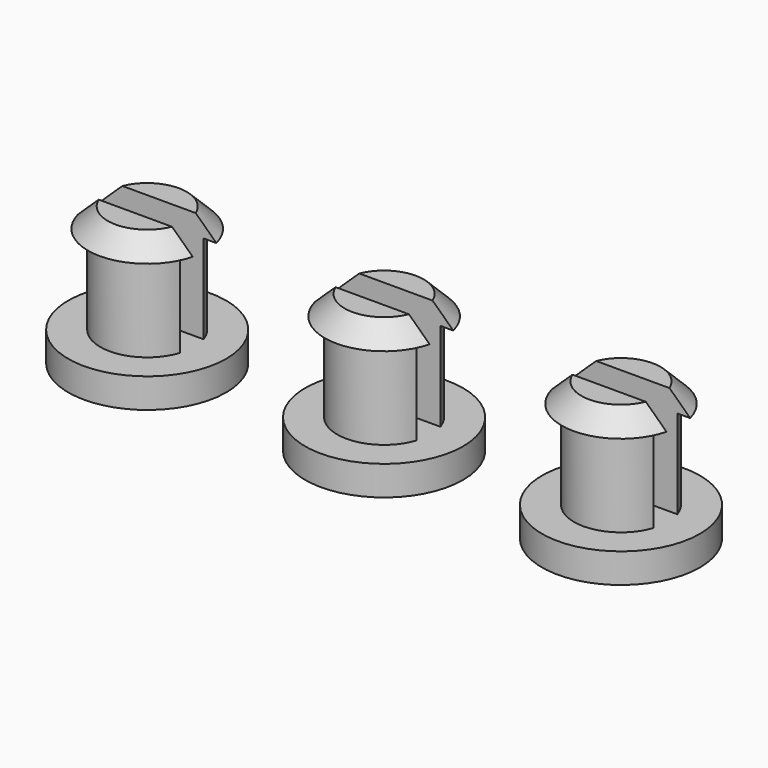
from build123d import *

# Parameters (mm, degrees)
F0_R     = 4
F1_DEPTH = 1.5
F2_DEPTH = 6.5
F3_START = 6
F3_DEPTH = 1
F4_SIZE  = 0.99999


# Not quite as in the source:
# - a fillet or chamfer is up to 0.001 mm smaller than in the source, because OpenCascade refuses the exact size


with BuildPart() as f1:
    # F0 (on Top) → F1 (new body)
    with BuildSketch(Plane.XY):
        Circle(F0_R)
        with BuildLine():
            ThreePointArc((-2.9047375097, 0.75), (0, 3), (2.9047375097, 0.75))
            Line((2.9047375097, 0.75), (3.5, 0.75))
            Line((3.5, 0.75), (3.5, -0.75))
            Line((3.5, -0.75), (2.9047375097, -0.75))
            ThreePointArc((2.9047375097, -0.75), (0, -3), (-2.9047375097, -0.75))
            Line((-2.9047375097, -0.75), (-3.5, -0.75))
            Line((-3.5, -0.75), (-3.5, 0.75))
            Line((-3.5, 0.75), (-2.9047375097, 0.75))
        make_face(mode=Mode.SUBTRACT)
        with BuildLine():
            ThreePointArc((2.2534695472, -0.75), (2.3444205227, -0.379891317), (2.375, 0))
            ThreePointArc((2.375, 0), (2.3444205227, 0.379891317), (2.2534695472, 0.75))
            Line((2.2534695472, 0.75), (-2.2534695472, 0.75))
            ThreePointArc((-2.2534695472, 0.75), (-2.375, 0), (-2.2534695472, -0.75))
            Line((-2.2534695472, -0.75), (2.2534695472, -0.75))
        make_face()
        with BuildLine():
            ThreePointArc((-2.2534695472, -0.75), (0, -2.375), (2.2534695472, -0.75))
            Line((2.2534695472, -0.75), (-2.2534695472, -0.75))
        make_face()
        with BuildLine():
            Line((-2.2534695472, 0.75), (2.2534695472, 0.75))
            ThreePointArc((2.2534695472, 0.75), (0, 2.375), (-2.2534695472, 0.75))
        make_face()
        with BuildLine():
            Line((2.9047375097, -0.75), (2.2534695472, -0.75))
            ThreePointArc((2.2534695472, -0.75), (0, -2.375), (-2.2534695472, -0.75))
            Line((-2.2534695472, -0.75), (-2.9047375097, -0.75))
            ThreePointArc((-2.9047375097, -0.75), (0, -3), (2.9047375097, -0.75))
        make_face()
        with BuildLine():
            ThreePointArc((-2.2534695472, 0.75), (0, 2.375), (2.2534695472, 0.75))
            Line((2.2534695472, 0.75), (2.9047375097, 0.75))
            ThreePointArc((2.9047375097, 0.75), (0, 3), (-2.9047375097, 0.75))
            Line((-2.9047375097, 0.75), (-2.2534695472, 0.75))
        make_face()
        with BuildLine():
            ThreePointArc((-2.2534695472, -0.75), (-2.375, 0), (-2.2534695472, 0.75))
            Line((-2.2534695472, 0.75), (-2.9047375097, 0.75))
            ThreePointArc((-2.9047375097, 0.75), (-3, 0), (-2.9047375097, -0.75))
            Line((-2.9047375097, -0.75), (-2.2534695472, -0.75))
        make_face()
        with BuildLine():
            ThreePointArc((2.2534695472, 0.75), (2.3444205227, 0.379891317), (2.375, 0))
            ThreePointArc((2.375, 0), (2.3444205227, -0.379891317), (2.2534695472, -0.75))
            Line((2.2534695472, -0.75), (2.9047375097, -0.75))
            ThreePointArc((2.9047375097, -0.75), (2.9760890888, -0.3780128774), (3, 0))
            ThreePointArc((3, 0), (2.9760890888, 0.3780128774), (2.9047375097, 0.75))
            Line((2.9047375097, 0.75), (2.2534695472, 0.75))
        make_face()
        with BuildLine():
            Line((3.5, 0.75), (2.9047375097, 0.75))
            ThreePointArc((2.9047375097, 0.75), (2.9760890888, 0.3780128774), (3, 0))
            ThreePointArc((3, 0), (2.9760890888, -0.3780128774), (2.9047375097, -0.75))
            Line((2.9047375097, -0.75), (3.5, -0.75))
            Line((3.5, -0.75), (3.5, 0.75))
        make_face()
        with BuildLine():
            ThreePointArc((-2.9047375097, -0.75), (-3, 0), (-2.9047375097, 0.75))
            Line((-2.9047375097, 0.75), (-3.5, 0.75))
            Line((-3.5, 0.75), (-3.5, -0.75))
            Line((-3.5, -0.75), (-2.9047375097, -0.75))
        make_face()
    extrude(amount=F1_DEPTH)

    # F0 (on Top) → F2 (join)
    with BuildSketch(Plane.XY):
        with BuildLine():
            Line((-2.2534695472, 0.75), (2.2534695472, 0.75))
            ThreePointArc((2.2534695472, 0.75), (0, 2.375), (-2.2534695472, 0.75))
        make_face()
        with BuildLine():
            ThreePointArc((-2.2534695472, -0.75), (0, -2.375), (2.2534695472, -0.75))
            Line((2.2534695472, -0.75), (-2.2534695472, -0.75))
        make_face()
    extrude(amount=F2_DEPTH)

    # F0 (on Top) → F3 (join)
    with BuildSketch(Plane.XY.offset(F3_START)):
        with BuildLine():
            Line((2.9047375097, -0.75), (2.2534695472, -0.75))
            ThreePointArc((2.2534695472, -0.75), (0, -2.375), (-2.2534695472, -0.75))
            Line((-2.2534695472, -0.75), (-2.9047375097, -0.75))
            ThreePointArc((-2.9047375097, -0.75), (0, -3), (2.9047375097, -0.75))
        make_face()
        with BuildLine():
            ThreePointArc((-2.2534695472, 0.75), (0, 2.375), (2.2534695472, 0.75))
            Line((2.2534695472, 0.75), (2.9047375097, 0.75))
            ThreePointArc((2.9047375097, 0.75), (0, 3), (-2.9047375097, 0.75))
            Line((-2.9047375097, 0.75), (-2.2534695472, 0.75))
        make_face()
        with BuildLine():
            Line((-2.2534695472, 0.75), (2.2534695472, 0.75))
            ThreePointArc((2.2534695472, 0.75), (0, 2.375), (-2.2534695472, 0.75))
        make_face()
        with BuildLine():
            ThreePointArc((-2.2534695472, -0.75), (0, -2.375), (2.2534695472, -0.75))
            Line((2.2534695472, -0.75), (-2.2534695472, -0.75))
        make_face()
    extrude(amount=F3_DEPTH)

    # F4 (size 1 in the source; OpenCascade refuses exactly that, so slightly less here)
    f4_edges = [f1.edges().sort_by_distance(p)[0] for p in [
        (0, 3, 7),
        (0, -3, 7),
    ]]
    chamfer(f4_edges, length=F4_SIZE)


with BuildPart() as f5_1:
    # F5: copy of F1
    add(f1.part.moved(Location((12, 0, 0))))


with BuildPart() as f6_1:
    # F6: copy of F1
    add(f1.part.moved(Location((24, 0, 0))))


solid = Compound([f1.part, f5_1.part, f6_1.part])
